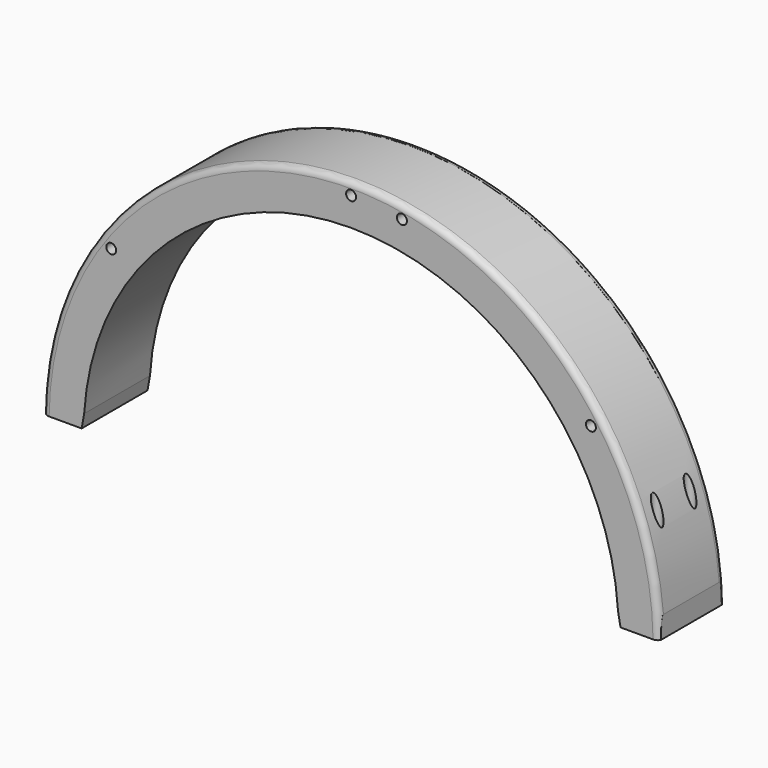
from build123d import *

# Parameters (mm, degrees)
F1_DEPTH    = 13
F2_D        = 1.57
F2_DEPTH    = 14.5
F2_TIP      = 0.4716755859
F4_D        = 3.5
F4_DEPTH    = 20
F4_TIP      = 1.0515060833
F6_D        = 1.57
F6_DEPTH    = 20
F6_TIP      = 0.4716755859
F7_T2_ANGLE = 185.2073223924
F7_T4_ANGLE = 185.2073223924


# Not quite as in the source:
# - a fillet or chamfer that OpenCascade refuses, or shapes differently, is made with other operations: its cross-section is extruded or revolved along the edge and cut away or added
# - a feature names something its author has since deleted; it is built from what else it names


with BuildPart() as f1:
    # F0 (on Front) → F1 (new body)
    with BuildSketch(Plane.XZ):
        with BuildLine():
            Line((-48.5584606546, 0.5), (-42.561347313, 0.5))
            Line((-42.561347313, 0.5), (-42.1642787203, 2.69))
            ThreePointArc((-42.1642787203, 2.69), (0, 42.25), (42.1642787203, 2.69))
            Line((42.1642787203, 2.69), (42.5584631857, 0.515907173))
            Line((42.5584631857, 0.515907173), (46.7514210343, 0.515907173))
            Line((46.7514210343, 0.515907173), (48.5457186432, 0.515907173))
            Line((48.5457186432, 0.515907173), (48.5457186432, 3.8733966245))
            ThreePointArc((48.5457186432, 3.8733966245), (-0.0818255025, 48.6999312585), (-48.5584606546, 3.7102424258))
            Line((-48.5584606546, 3.7102424258), (-48.5584606546, 0.5))
        make_face()
    extrude(amount=F1_DEPTH)

    # F2
    with Locations(Plane(origin=(0, 0, 0), x_dir=(1, 0, 0), z_dir=(0, 1, 0))):
        with Locations((0, -46.75), (8.0312282171, -46.0473585768), (37.8857820484, -27.0279101812), (-37.8857820484, -27.0279101812)):
            Hole(F2_D / 2, depth=F2_DEPTH)
            with Locations((0, 0, -(F2_DEPTH + F2_TIP / 2))):  # 118° drill point
                Cone(0, F2_D / 2, F2_TIP, mode=Mode.SUBTRACT)

    # F4
    with Locations(Plane(origin=(0, 0, 0.5), x_dir=(1, 0, 0), z_dir=(0, 0, -1))):
        with Locations((-45.7584606546, 9.75), (-45.7584606546, 3.25)):
            Hole(F4_D / 2, depth=F4_DEPTH)
            with Locations((0, 0, -(F4_DEPTH + F4_TIP / 2))):  # 118° drill point
                Cone(0, F4_D / 2, F4_TIP, mode=Mode.SUBTRACT)

    # F6
    with Locations(Plane(origin=(0, 0, 0.515907173), x_dir=(1, 0, 0), z_dir=(0, 0, -1))):
        with Locations((45.7457186432, 3.25), (45.7457186432, 9.75)):
            Hole(F6_D / 2, depth=F6_DEPTH)
            with Locations((0, 0, -(F6_DEPTH + F6_TIP / 2))):  # 118° drill point
                Cone(0, F6_D / 2, F6_TIP, mode=Mode.SUBTRACT)

    # F7: fillet of radius 1 on 2 edges, made by hand

    # F7_s1 → F7_t2 (revolve, cut)
    with BuildSketch(Plane(origin=(0, 0, 0), x_dir=(0, 1, 0), z_dir=(-0.0437482975, 0, -0.9990425849))):
        with BuildLine():
            ThreePointArc((-12, 48.7), (-12.7071067812, 48.4071067812), (-13, 47.7))
            Line((-13, 47.7), (-13.02, 47.7))
            Line((-13.02, 47.7), (-13.02, 48.72))
            Line((-13.02, 48.72), (-12, 48.72))
            Line((-12, 48.72), (-12, 48.7))
        make_face()
    revolve(axis=Axis((0, -13, 0), (0, -1, 0)), revolution_arc=F7_T2_ANGLE, mode=Mode.SUBTRACT)

    # F7_s3 → F7_t4 (revolve, cut)
    with BuildSketch(Plane(origin=(0, 0, 0), x_dir=(0, 1, 0), z_dir=(-0.0437482975, 0, -0.9990425849))):
        with BuildLine():
            ThreePointArc((-1, 48.7), (-0.2928932188, 48.4071067812), (0, 47.7))
            Line((0, 47.7), (0.02, 47.7))
            Line((0.02, 47.7), (0.02, 48.72))
            Line((0.02, 48.72), (-1, 48.72))
            Line((-1, 48.72), (-1, 48.7))
        make_face()
    revolve(axis=Axis((0, 0, 0), (0, -1, 0)), revolution_arc=F7_T4_ANGLE, mode=Mode.SUBTRACT)


solid = f1.part
